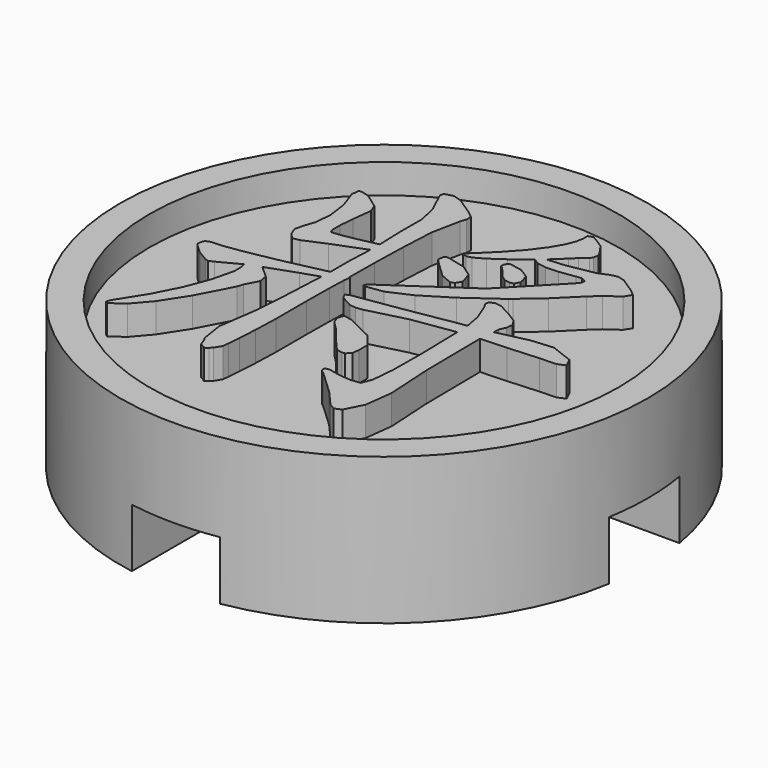
from build123d import *

# Parameters (mm, degrees)
F0_R     = 9
F1_DEPTH = 4
F3_W     = 3
F3_H     = 3
F4_DEPTH = 2
F2_R     = 9
F2_R_2   = 8
F5_DEPTH = 1
F7_DEPTH = 1


# Not quite as in the source:
# - a feature names something its author has since deleted; it is built from what else it names


with BuildPart() as f1:
    # F0 (on Top) → F1 (new body)
    with BuildSketch(Plane.XY):
        with Locations((-31.3306450844, 19.7580661625)):
            Circle(F0_R)
    extrude(amount=F1_DEPTH)

    # F3 (on face) → F4 (cut)
    with BuildSketch(Plane(origin=(0, 0, 0), x_dir=(1, 0, 0), z_dir=(0, 0, -1))):
        with BuildLine():
            ThreePointArc((-32.8306450844, -28.6321858371), (-32.0832814269, -28.7265408676), (-31.3306450844, -28.7580661625))
            ThreePointArc((-31.3306450844, -28.7580661625), (-30.5780087419, -28.7265408676), (-29.8306450844, -28.6321858371))
            Line((-29.8306450844, -28.6321858371), (-29.8306450844, -21.2580661625))
            Line((-29.8306450844, -21.2580661625), (-32.8306450844, -21.2580661625))
            Line((-32.8306450844, -21.2580661625), (-32.8306450844, -28.6321858371))
        make_face()
        with BuildLine():
            ThreePointArc((-40.204764759, -18.2580661625), (-40.2991197895, -19.0054298199), (-40.3306450844, -19.7580661625))
            ThreePointArc((-40.3306450844, -19.7580661625), (-40.2991197895, -20.510702505), (-40.204764759, -21.2580661625))
            Line((-40.204764759, -21.2580661625), (-32.8306450844, -21.2580661625))
            Line((-32.8306450844, -21.2580661625), (-32.8306450844, -18.2580661625))
            Line((-32.8306450844, -18.2580661625), (-40.204764759, -18.2580661625))
        make_face()
        with Locations((-31.3306450844, -19.7580661625)):
            Rectangle(F3_W, F3_H)
        with BuildLine():
            Line((-29.8306450844, -18.2580661625), (-29.8306450844, -21.2580661625))
            Line((-29.8306450844, -21.2580661625), (-22.4565254097, -21.2580661625))
            ThreePointArc((-22.4565254097, -21.2580661625), (-22.3621703793, -20.510702505), (-22.3306450844, -19.7580661625))
            ThreePointArc((-22.3306450844, -19.7580661625), (-22.3621703793, -19.0054298199), (-22.4565254097, -18.2580661625))
            Line((-22.4565254097, -18.2580661625), (-29.8306450844, -18.2580661625))
        make_face()
        with BuildLine():
            Line((-32.8306450844, -10.8839464878), (-32.8306450844, -18.2580661625))
            Line((-32.8306450844, -18.2580661625), (-29.8306450844, -18.2580661625))
            Line((-29.8306450844, -18.2580661625), (-29.8306450844, -10.8839464878))
            ThreePointArc((-29.8306450844, -10.8839464878), (-30.5780087419, -10.7895914574), (-31.3306450844, -10.7580661625))
            ThreePointArc((-31.3306450844, -10.7580661625), (-32.0832814269, -10.7895914574), (-32.8306450844, -10.8839464878))
        make_face()
    extrude(amount=-F4_DEPTH, mode=Mode.SUBTRACT)

    # F2 (on face) → F5 (join)
    with BuildSketch(Plane.XY.offset(4)):
        with Locations((-31.3306450844, 19.7580661625)):
            Circle(F2_R)
        with Locations((-31.3306450844, 19.7580661625)):
            Circle(F2_R_2, mode=Mode.SUBTRACT)
    extrude(amount=F5_DEPTH)

    # F6 (on face) → F7 (join)
    with BuildSketch(Plane.XY.offset(4)):
        Polygon((-36.2666520069, 18.698154303), (-35.559345186, 19.0707798106), (-35.5127693448, 18.9069099648), (-35.5075928604, 18.6153430708), (-35.6921811626, 17.8545688617), (-36.0009800537, 17.0437761676), (-36.4434724528, 16.1777509479), (-37.0291537973, 15.2479116305), (-37.0843581557, 15.09955246), (-37.0050033379, 15.047793875), (-36.5633703479, 15.3591841381), (-36.0570450732, 15.9483143858), (-35.4989674727, 16.8134632961), (-34.9038032094, 17.9494543847), (-34.8356576398, 18.160795159), (-34.6105400309, 18.5912132673), (-34.6622735784, 18.8844764458), (-35.079766124, 19.2571019534), (-34.0869639809, 19.6090152639), (-33.4995487958, 19.8056966349), (-33.5487222682, 18.7913122447), (-33.5892640937, 17.9813583038), (-33.633248563, 17.3620579776), (-33.6893135824, 16.9178192193), (-33.8402641248, 15.8741285412), (-33.7410721674, 15.2203078865), (-33.7100070014, 15.0874719099), (-33.6479142256, 14.9787907742), (-33.5754622216, 14.7657411967), (-33.4477902108, 14.6993232084), (-33.3856911756, 14.6441157202), (-33.2718398149, 14.7269206931), (-33.1855671608, 14.8140446191), (-33.0475609591, 15.047793875), (-33.0277313307, 15.2496392118), (-32.992353471, 15.6679767699), (-32.9552793267, 16.3011040056), (-32.9268180514, 17.1455469782), (-32.9276755827, 18.4523370156), (-32.9173226138, 19.4106376083), (-32.897467948, 20.0092445155), (-32.8716105632, 20.23353589), (-32.8992143073, 20.2473064653), (-32.8897188697, 21.3022577183), (-32.8578086912, 22.5072456484), (-32.8008611031, 23.6311749649), (-32.6059260914, 24.6015623671), (-32.5446908469, 24.7843980506), (-32.5369229905, 24.9776242591), (-32.8077714281, 25.1846210429), (-33.3546447878, 25.5503550035), (-33.6504993382, 25.6409278327), (-33.9273755321, 25.5641881723), (-33.9661960357, 25.4503305522), (-33.9032206912, 25.298478663), (-33.6073724002, 24.6619025242), (-33.4753876955, 24.042602198), (-33.4797191674, 23.1420691686), (-33.4477902108, 22.2277655638), (-34.105066028, 22.0854278903), (-34.5579176552, 22.0043692768), (-34.8235833491, 21.9715702702), (-34.9176050814, 21.9724465795), (-34.9615895507, 22.1027037029), (-34.9615895507, 22.4226817975), (-34.920190194, 22.921239216), (-34.8382427524, 23.5871717175), (-34.9452088255, 23.8648991834), (-35.4523916316, 24.2288805253), (-35.683555775, 24.2849643228), (-35.8146641703, 24.2944785385), (-35.8388190112, 24.0149984539), (-35.6231780617, 23.4034597247), (-35.5317477013, 22.7211277198), (-35.5852276081, 22.1553448566), (-35.7077106159, 21.7861056587), (-35.7767137167, 21.5066881676), (-35.6801068718, 21.2513065898), (-35.4955185696, 21.0434334967), (-35.2660757481, 21.0891893627), (-34.5380692488, 21.3997158352), (-33.4477902108, 21.8240999277), (-33.4857469237, 20.9865359834), (-33.4857469237, 20.1679691736), (-34.8874224842, 19.8609041231), (-35.9414598718, 19.6564736738), (-36.6608397316, 19.5477862787), (-37.0567562895, 19.526210291), (-37.1964913243, 19.4736129528), (-37.2430696692, 19.3916655112), (-37.2637712254, 19.2225878843), (-37.1775148456, 19.1259810394), (-36.9144336384, 18.8844764458), (-36.5357666039, 18.6567486869), (-36.4305343714, 18.625702299), align=None)
        Polygon((-31.6898949054, 22.5150072454), (-31.6019197075, 22.4141064847), (-31.0205573161, 21.8594652688), (-30.6254669928, 21.692966495), (-30.4943961536, 21.738722361), (-30.3839811773, 21.9310722602), (-30.4357460216, 22.1139079437), (-30.5185572538, 22.3450658278), (-30.9075134118, 22.6142179809), (-31.5605140913, 22.7728925641), (-31.6674551271, 22.7392798418), (-31.6812569991, 22.6279885561), align=None)
        Polygon((-30.1528232933, 23.2714499826), (-30.0631267734, 23.2111098255), (-29.7456524198, 22.8281000523), (-29.5680119988, 22.6909576413), (-29.3730331716, 22.6659202317), (-29.2454049762, 22.6927102599), (-29.1591511001, 22.8660317278), (-29.1850022256, 23.0058030669), (-29.2660608391, 23.2248804008), (-29.599934696, 23.4318771846), (-30.0389656731, 23.5078031291), (-30.1458754121, 23.3870602214), align=None)
        Polygon((-30.2528477446, 23.6811871906), (-29.6662838314, 24.1219707864), (-29.4938386728, 23.99947526), (-29.1806832724, 23.948586725), (-28.7468475577, 23.9649862283), (-28.2102958702, 24.042602198), (-28.0162559459, 24.0633206544), (-27.8618377222, 23.9873947098), (-27.8739182724, 23.8640854676), (-27.98258063, 23.7217477941), (-29.6369900622, 22.0130071831), (-32.2160560679, 20.2473064653), (-32.3333751099, 20.1282911388), (-32.2436535527, 20.0886068446), (-31.6562383676, 20.1722756081), (-30.8851049302, 20.5164586184), (-29.9354359845, 21.1012699129), (-28.8106303587, 21.9069111599), (-28.717491195, 21.9862797483), (-28.0024227771, 22.6029511466), (-27.2752738091, 23.3180195644), (-26.9561720238, 23.6130228429), (-26.5128220935, 23.9218592902), (-26.3644128482, 24.1599024619), (-26.5757285851, 24.3367291671), (-27.0855528379, 24.6705404305), (-27.3261623441, 24.7335095156), (-27.5547538936, 24.6843110058), (-27.891194085, 24.5420359258), (-28.2620607145, 24.4704289344), (-28.872785728, 24.3626428861), (-29.4386311847, 24.3220822825), (-29.2574855263, 24.5040416567), (-29.0108044483, 24.7223052748), (-28.8244635275, 24.9172215085), (-28.5967482872, 25.0983671669), (-28.5337792021, 25.1923826399), (-28.5036091236, 25.3640140826), (-28.5881103809, 25.5210612343), (-28.7968597834, 25.8194445631), (-29.0651356271, 25.9945812432), (-29.2660608391, 26.1127578164), (-29.4325596129, 26.0523550658), (-29.4247980159, 25.8712094074), (-29.4688012633, 25.6254046387), (-29.5990583866, 25.3027976162), (-29.8354115332, 24.9008220052), (-30.1976402564, 24.4152214462), (-30.6591423087, 23.9089024308), (-31.1602848397, 23.4112213216), (-31.3362352356, 23.2524841448), (-31.3448668825, 23.1532734093), (-31.2292941999, 23.1317412371), (-31.051603704, 23.1696729126), (-30.7203587751, 23.3577038586), align=None)
        Polygon((-30.133794862, 19.3433558294), (-28.6761168756, 19.564167004), (-28.6398752253, 17.9598073535), (-28.6519557754, 16.7850020207), (-28.720120123, 16.0276641961), (-28.8520672715, 15.6757383669), (-29.1729216754, 15.6343390102), (-29.5835351927, 15.6697043512), (-29.9699250162, 15.755100696), (-30.1131389991, 15.7326734363), (-30.1321048368, 15.6757383669), (-30.1070674272, 15.579131522), (-29.9699250162, 15.4756268708), (-29.1884448694, 14.743313937), (-28.7037206197, 14.1921341429), (-28.4975375517, 14.0713749609), (-28.2758938833, 14.1645322767), (-27.9679337454, 14.7717752124), (-27.848067147, 15.7274969519), (-27.9420200264, 17.3430671025), (-27.9688100547, 19.6469782362), (-27.0794812661, 19.686656271), (-26.029787869, 19.7539380499), (-25.4656324374, 19.7737676783), (-25.2016755468, 19.8850401859), (-25.3500847922, 20.1817710457), (-26.1074038387, 20.4741453962), (-26.8578375977, 20.4094862859), (-27.9170452104, 20.1679691736), (-27.9067172789, 20.3827588511), (-27.8100728779, 20.581994038), (-27.7876643963, 20.8140282313), (-27.9273731418, 21.0236539431), (-28.3241534903, 21.2746539743), (-28.7037206197, 21.4652512548), (-28.9331258851, 21.4988639772), (-29.0797825117, 21.4376475107), (-29.1177141873, 21.3117093405), (-29.0108044483, 21.1305636821), (-28.7942934489, 20.5733561317), (-28.6898874509, 20.0196037437), (-29.0384081924, 19.9678451588), (-30.5832163641, 19.7047645775), (-32.2298516806, 19.4468729994), (-32.3730343667, 19.3813125424), (-32.2850591688, 19.2191452404), (-31.895182886, 19.0052381316), (-31.6786781459, 18.975919325), (-31.4431950494, 19.0052381316), align=None)
        Polygon((-31.6122538983, 17.9899962101), (-31.3465882045, 17.7217454038), (-30.7048355812, 16.9454229633), (-30.5418420448, 16.7712001487), (-30.3460495018, 16.7315221139), (-30.2416435038, 16.7427388734), (-30.1045010927, 16.8902217345), (-30.0768973487, 17.1153643809), (-30.0768973487, 17.4940176449), (-30.4365597374, 17.926157075), (-31.3224333636, 18.3634855084), (-31.6157215795, 18.4152440933), (-31.6812569991, 18.2013182064), align=None)
    extrude(amount=F7_DEPTH)


solid = f1.part
